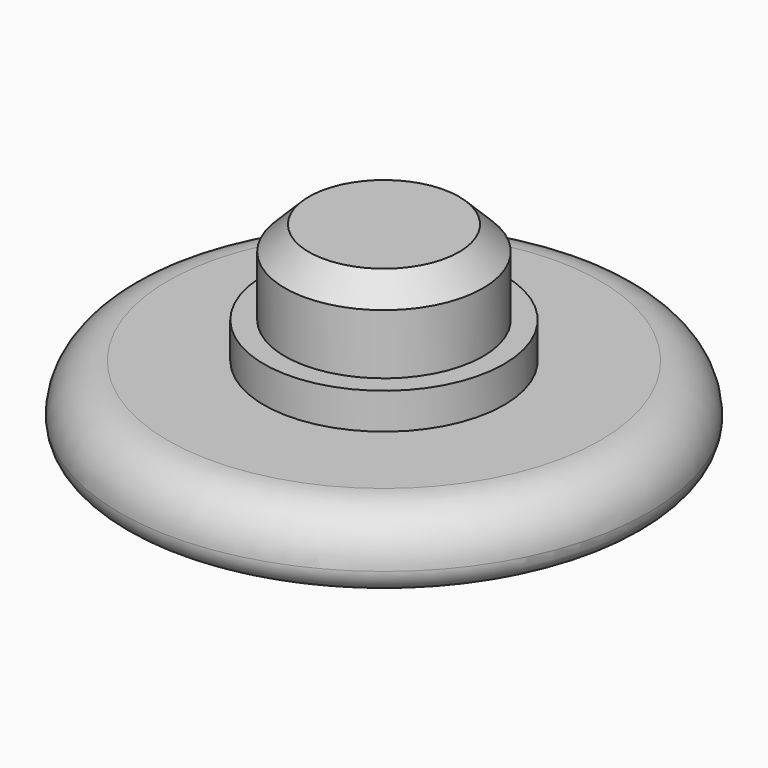
from build123d import *

# Parameters (mm, degrees)
F1_R     = 11
F1_R_2   = 5
F1_R_3   = 4.125
F2_DEPTH = 3
F3_START = 2
F3_DEPTH = 6
F4_START = 3
F4_DEPTH = 1.5
F5_SIZE  = 1
F6_R     = 1
F7_R     = 1.99999


# Not quite as in the source:
# - a fillet or chamfer that OpenCascade refuses, or shapes differently, is made with other operations: its cross-section is extruded or revolved along the edge and cut away or added
# - a fillet or chamfer is up to 0.001 mm smaller than in the source, because OpenCascade refuses the exact size


with BuildPart() as f2:
    # F1 (on Top) → F2 (new body)
    with BuildSketch(Plane.XY):
        Circle(F1_R)
        Circle(F1_R_2, mode=Mode.SUBTRACT)
        Circle(F1_R_2)
        Circle(F1_R_3, mode=Mode.SUBTRACT)
    extrude(amount=F2_DEPTH)

    # F1 (on Top) → F3 (join)
    with BuildSketch(Plane.XY.offset(F3_START)):
        Circle(F1_R_3)
    extrude(amount=F3_DEPTH)

    # F1 (on Top) → F4 (join)
    with BuildSketch(Plane.XY.offset(F4_START)):
        Circle(F1_R_2)
        Circle(F1_R_3, mode=Mode.SUBTRACT)
    extrude(amount=F4_DEPTH)

    # F5
    f5_edges = [f2.edges().sort_by_distance(p)[0] for p in [
        (-4.125, 0, 8),
    ]]
    chamfer(f5_edges, length=F5_SIZE)

    # F6
    f6_edges = [f2.edges().sort_by_distance(p)[0] for p in [
        (-11, 0, 0),
    ]]
    fillet(f6_edges, radius=F6_R)

    # F7 (radius 2 in the source; OpenCascade refuses exactly that, so slightly less here)
    f7_edges = [f2.edges().sort_by_distance(p)[0] for p in [
        (-11, 0, 3),
    ]]
    fillet(f7_edges, radius=F7_R)

    # F8: fillet of radius 8 on 1 edges, made by hand

    # F8_s1 → F8_t2 (revolve, cut)
    with BuildSketch(Plane.XZ):
        with BuildLine():
            ThreePointArc((9.4165026221, 0), (6.5880754974, 0.5166852265), (4.125, 2))
            Line((4.125, 2), (4.0191699476, 1.88))
            ThreePointArc((4.0191699476, 1.88), (3.965, 1), (3.965, 0))
            Line((3.965, 0), (4.125, -0.16))
            Line((4.125, -0.16), (9.4165026221, -0.16))
            Line((9.4165026221, -0.16), (9.4165026221, 0))
        make_face()
    revolve(axis=Axis((0, 0, 0), (0, 0, 1)), mode=Mode.SUBTRACT)


solid = f2.part
